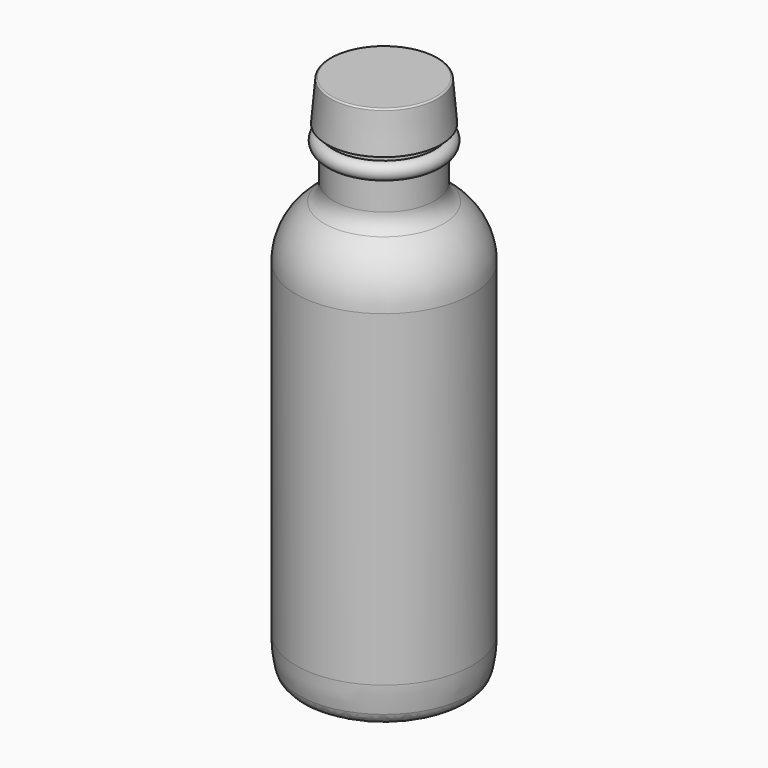
from build123d import *

# Parameters (mm, degrees)
F2_R = 5.08
F3_T = 2.54
F6_R = 0.508


# Not quite as in the source:
# - a shell that OpenCascade refuses in one call is made with other operations: the cavity is built on its own and cut out


with BuildPart() as f1:
    # F0 (on Front) → F1 (revolve)
    with BuildSketch(Plane.XZ):
        with BuildLine():
            Line((0, 152.4), (0, 0))
            Line((0, 0), (25.4, 0))
            ThreePointArc((25.4, 0), (26.8828082767, 6.1516598374), (27.3812, 12.4598485497))
            Line((27.3812, 12.4598485497), (27.3812, 114.0598485497))
            ThreePointArc((27.3812, 114.0598485497), (25.0414004497, 123.390348849), (18.5757340104, 130.5127118886))
            ThreePointArc((18.5757340104, 130.5127118886), (16.4993890547, 132.7999444127), (15.748, 135.796284761))
            Line((15.748, 135.796284761), (15.748, 144.7801431968))
            ThreePointArc((15.748, 144.7801431968), (18.3070713092, 147.3200715984), (15.748, 149.86))
            Line((15.748, 149.86), (15.748, 152.4))
            Line((15.748, 152.4), (0, 152.4))
        make_face()
    revolve(axis=Axis((0, 0, 76.2), (0, 0, -1)))

    # F2
    f2_edges = [f1.edges().sort_by_distance(p)[0] for p in [
        (-25.4, 0, 0),
    ]]
    fillet(f2_edges, radius=F2_R)

    # F3: shell of thickness 2.54, made by hand


with BuildPart() as f3_core1:
    # F3_t2: copy of F1
    add(f1.part)

    # the walls: a layer under each face that stays
    f3_faces = [f3_core1.faces().sort_by_distance(p)[0] for p in [
        (0, 0, 0),
        (-24.7085178809, 0, 1.1281862172),
        (-27.1559674596, 0, 8.2119271912),
        (-27.3812, 0, 63.2598485497),
        (-25.0414004497, 0, 123.390348849),
        (-16.4993890547, 0, 132.7999444127),
        (-15.748, 0, 140.2882139789),
        (-15.748, 0, 151.13),
    ]]
    thicken(f3_faces, amount=-F3_T, mode=Mode.SUBTRACT)

    # F3_s3 → F3_t4 (revolve, cut)
    with BuildSketch(Plane.XZ):
        Polygon((15.7732092869, 144.7547439128), (13.208, 144.7801431968), (13.208, 147.3392866441), (15.7670713092, 147.3200715984), align=None)
    revolve(axis=Axis((0, 0, 144.7801431968), (0, 0, -1)), mode=Mode.SUBTRACT)

    # F3_s5 → F3_t6 (revolve, cut)
    with BuildSketch(Plane.XZ):
        Polygon((15.7732092869, 149.885399284), (15.7670713092, 147.3200715984), (13.208, 147.3008565527), (13.208, 149.86), align=None)
    revolve(axis=Axis((0, 0, 149.86), (0, 0, -1)), mode=Mode.SUBTRACT)


with BuildPart() as f1_1:
    add(f1.part)

    # what is left inside the walls is the cavity
    f3_cavity = [f3_core1.part.solids().sort_by_distance(p)[0] for p in [
        (-24.8158, 0, 46.326515),
    ]]
    add(f3_cavity, mode=Mode.SUBTRACT)

    # F4 (on Front) → F5 (revolve)
    with BuildSketch(Plane.XZ):
        Polygon((0, 164.5454947654), (0, 151.892), (17.7546, 151.892), (16.66875, 164.5454947654), align=None)
    revolve(axis=Axis((0, 0, 158.2187473827), (0, 0, -1)))

    # F6
    f6_edges = [f1_1.edges().sort_by_distance(p)[0] for p in [
        (-16.66875, 0, 164.545495),
    ]]
    fillet(f6_edges, radius=F6_R)


solid = f1_1.part
